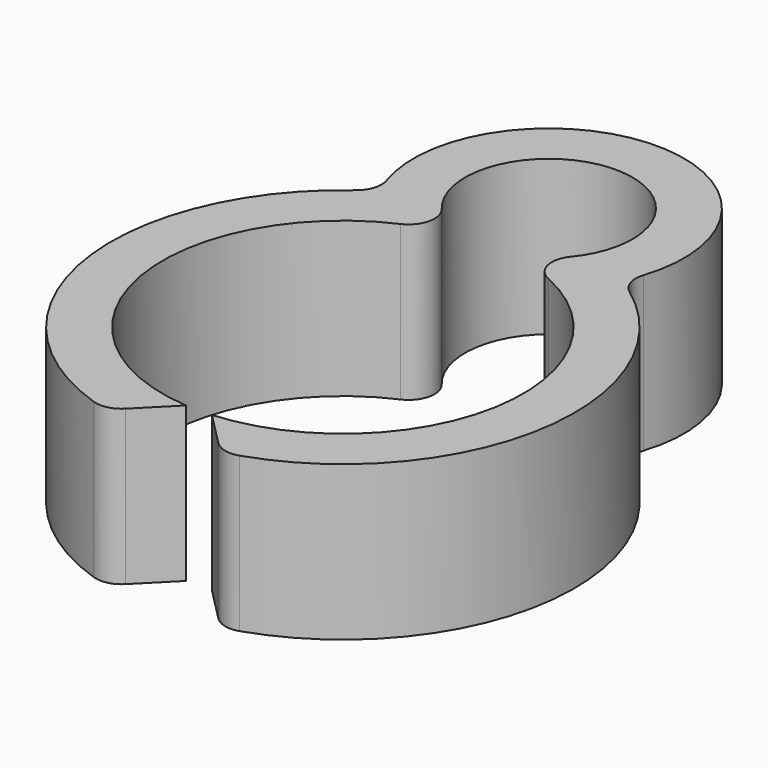
from build123d import *

# Parameters (mm, degrees)
F1_DEPTH = 6
F3_DEPTH = 6.001
F4_R     = 1


with BuildPart() as f1:
    # F0 (on Top) → F1 (new body)
    with BuildSketch(Plane.XY):
        with BuildLine():
            ThreePointArc((-4.7055641516, 7.671875), (0, -9), (4.7055641516, 7.671875))
            ThreePointArc((4.7055641516, 7.671875), (0, 15.25), (-4.7055641516, 7.671875))
        make_face()
        with BuildLine():
            ThreePointArc((1.0429029122, 6.921875), (0, -7), (-1.0429029122, 6.921875))
            ThreePointArc((-1.0429029122, 6.921875), (0, 13.25), (1.0429029122, 6.921875))
        make_face(mode=Mode.SUBTRACT)
    extrude(amount=F1_DEPTH)

    # F2 (on face) → F3 (cut, through all)
    with BuildSketch(Plane.XY.offset(6)):
        with BuildLine():
            ThreePointArc((0.5, -6.9821200219), (0, -7), (-0.5, -6.9821200219))
            Line((-0.5, -6.9821200219), (-2.2234871513, -8.7210151294))
            ThreePointArc((-2.2234871513, -8.7210151294), (-1.1204605827, -8.9299814156), (0, -9))
            ThreePointArc((0, -9), (1.1204605827, -8.9299814156), (2.2234871513, -8.7210151294))
            Line((2.2234871513, -8.7210151294), (0.5, -6.9821200219))
        make_face()
    extrude(amount=-F3_DEPTH, mode=Mode.SUBTRACT)

    # F4
    f4_edges = [f1.edges().sort_by_distance(p)[0] for p in [
        (-1.042903, 6.921875, 3),
        (4.705564, 7.671875, 3),
        (2.223487, -8.721015, 3),
        (-2.223487, -8.721015, 3),
        (-4.705564, 7.671875, 3),
        (1.042903, 6.921875, 3),
    ]]
    fillet(f4_edges, radius=F4_R)


solid = f1.part
